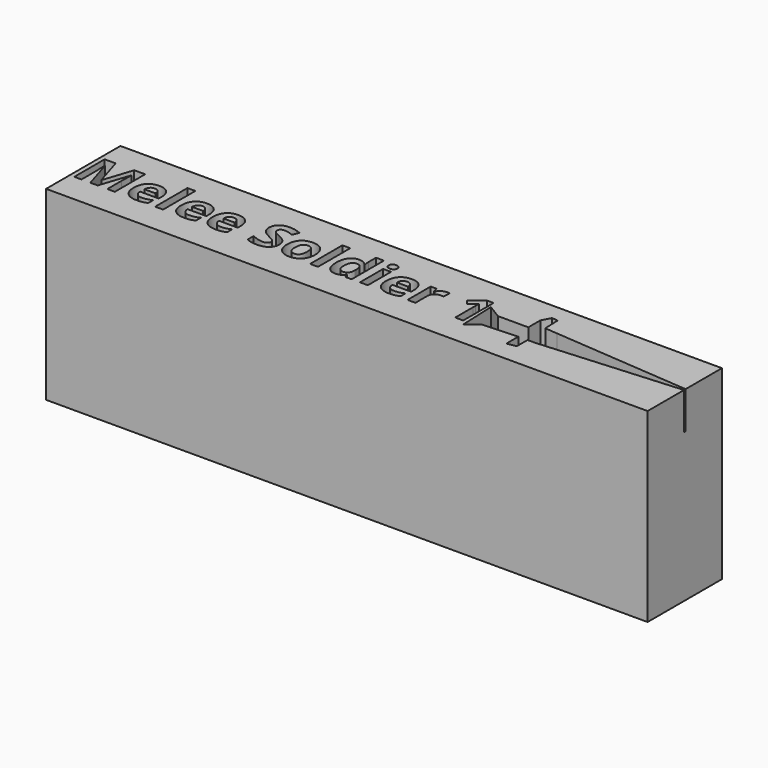
from build123d import *

# Parameters (mm, degrees)
F0_W         = 50.8
F0_H         = 6.35
F1_DEPTH     = 12.7
F2_W         = 6.35
F2_H         = 3.175
F3_DEPTH     = 25.4
F4_W         = 6.35
F4_H         = 3.6267349496
F4_H_2       = 3.9137584761
F5_DEPTH     = 25.4
F6_TEXT_SIZE = 3.6318438813
F7_DEPTH     = 2.54
F9_DEPTH     = 2.54
F10_W        = 1.2841656148
F10_H        = 6.35
F12_DEPTH    = 25.4
F14_DEPTH    = 25.4
F15_W        = 21.4077578858
F15_H        = 23.4408974648
F16_DEPTH    = 7.62


# Not quite as in the source:
# - Text() gives the source's letters only with a copy of the font that has no kerning and outlines rounded to 1/6400 em; it was checked with that copy


with BuildPart() as f1:
    # F0 (on Top) → F1 (new body)
    with BuildSketch(Plane.XY):
        Rectangle(F0_W, F0_H)
    extrude(amount=F1_DEPTH)

    # F2 (on face) → F3 (cut)
    with BuildSketch(Plane.XY.offset(12.7)):
        with Locations((22.225, -1.5875)):
            Rectangle(F2_W, F2_H)
    extrude(amount=-F3_DEPTH, mode=Mode.SUBTRACT)

    # F4 (on face) → F5 (cut)
    with BuildSketch(Plane.XZ):
        with Locations((22.225, 6.9728740491)):
            Rectangle(F4_W, F4_H)
        with Locations((22.225, 10.743120762)):
            Rectangle(F4_W, F4_H_2)
    extrude(amount=-F5_DEPTH, mode=Mode.SUBTRACT)

    # F6 (on face) → F7 (cut)
    with BuildSketch(Plane.XY.offset(12.7)):
        with Locations((-23.3615717152, -1.1490484467)):
            Text('Melee Soldier 1', F6_TEXT_SIZE, font='Open Sans', font_style=FontStyle.BOLD, text_align=(TextAlign.LEFT, TextAlign.BOTTOM))
    extrude(amount=-F7_DEPTH, mode=Mode.SUBTRACT)

    # F8 (on face) → F9 (cut)
    with BuildSketch(Plane.XY.offset(12.7)):
        Polygon((18.6902992427, 0), (8.3850220263, 0.8138253183), (7.5388358832, 0.8806500813), (7.5013757636, 1.7678158124), (7.491487857, 2.0019905008), (7.0790257305, 2.0345633384), (6.7592654377, 1.4293312127), (6.7592654377, 0.4050029092), (4.6870978549, 0.4050029092), (3.7359795533, 0.9833658203), (3.8405575548, -1.4933486205), (4.5675016008, -0.895549194), (7.0192278363, -0.775952707), (7.0192278363, -1.7925222637), (7.6471087523, -1.6835696836), (7.6471087523, -0.775952707), (8.2962800866, -0.7556193371), align=None)
    extrude(amount=-F9_DEPTH, mode=Mode.SUBTRACT)

    # F10 (on face) → F12 (cut)
    with BuildSketch(Plane.XY.offset(12.7)):
        with Locations((-24.7579171926, 0)):
            Rectangle(F10_W, F10_H)
    extrude(amount=-F12_DEPTH, mode=Mode.SUBTRACT)

    # F13 (on face) → F14 (cut)
    with BuildSketch(Plane.XY.offset(12.7)):
        Polygon((-24.1158343852, -3.175), (-23.3430471271, -3.175), (-23.3430471271, 3.175), (-23.3469232917, 3.175), (-24.1158343852, 3.175), align=None)
    extrude(amount=-F14_DEPTH, mode=Mode.SUBTRACT)

    # F15 (on face) → F16 (cut)
    with BuildSketch(Plane.YZ.offset(25.4)):
        with Locations((2.5316798128, 7.6622385532)):
            Rectangle(F15_W, F15_H)
    extrude(amount=-F16_DEPTH, mode=Mode.SUBTRACT)


solid = f1.part
